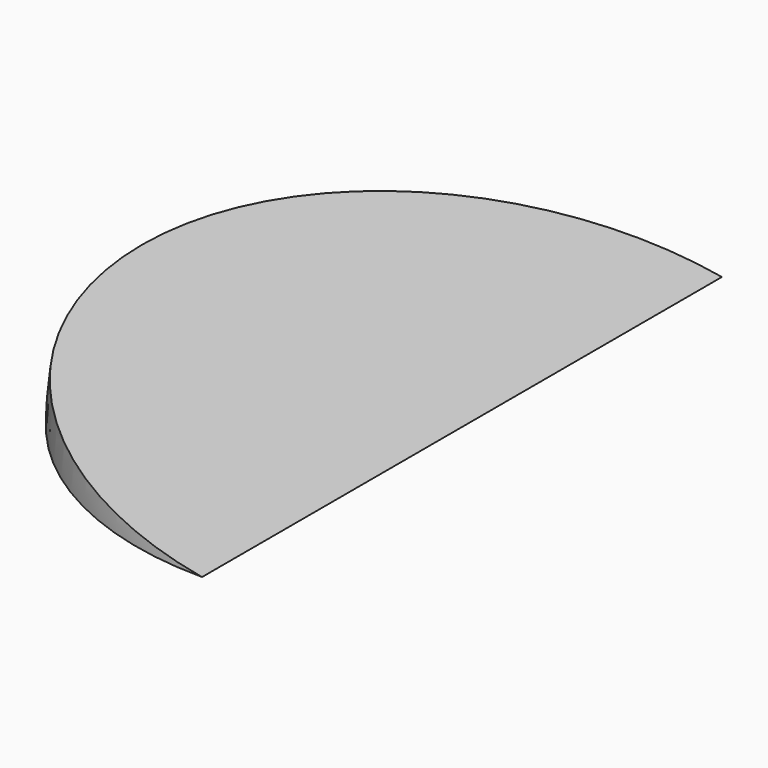
from build123d import *

# Parameters (mm, degrees)
F2_ANGLE = 10


# Not quite as in the source:
# - the program builds the solid bodies; features that only make, move or delete a surface that nothing else refers to are left out


with BuildPart() as f2:
    # F0 (on Top) → F2 (revolve)
    with BuildSketch(Plane.XY):
        with BuildLine():
            Line((0, 0), (0, 50.8))
            ThreePointArc((0, 50.8), (-50.8, 0), (0, -50.8))
            Line((0, -50.8), (0, 0))
        make_face()
    revolve(axis=Axis((0, -13.0201773718, 0), (0, 1, 0)), revolution_arc=F2_ANGLE)


solid = f2.part
